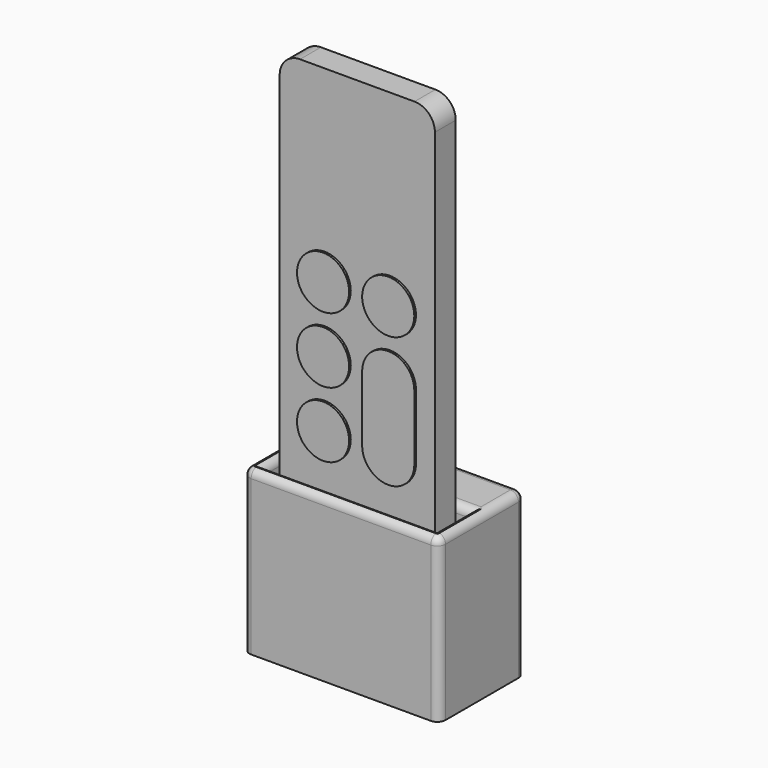
from build123d import *

# Parameters (mm, degrees)
F1_DEPTH      = 6.4
F2_R          = 6.4
F3_DEPTH      = 0.5
F5_DEPTH      = 35
F5_DEPTH_BACK = 5
F6_T          = -3
F7_W          = 48.1
F7_H          = 40
F8_DEPTH      = 10
F9_T1_DEPTH   = 22.4
F9_T3_DEPTH   = 44.1
F9_T5_DEPTH   = 10.4
F9_T7_DEPTH   = 42.1
F9_T9_DEPTH   = 43
F9_S13_W      = 2
F9_S13_H      = 2
F9_T14_DEPTH  = 2
F9_S19_W      = 2
F9_S19_H      = 2
F9_T20_DEPTH  = 2
F9_S25_W      = 2
F9_S25_H      = 2
F9_T26_DEPTH  = 2
F9_S31_W      = 2
F9_S31_H      = 2
F9_T32_DEPTH  = 2
F9_T39_DEPTH  = 15.4
F9_T43_DEPTH  = 47.1
F9_T50_DEPTH  = 15.4
F9_T54_DEPTH  = 47.1
F9_T61_DEPTH  = 47.1
F9_T65_DEPTH  = 15.4
F9_T72_DEPTH  = 15.4
F9_T76_DEPTH  = 47.1


# Not quite as in the source:
# - a fillet or chamfer that OpenCascade refuses, or shapes differently, is made with other operations: its cross-section is extruded or revolved along the edge and cut away or added


with BuildPart() as f1:
    # F0 (on Front) → F1 (new body)
    with BuildSketch(Plane.XZ):
        with BuildLine():
            ThreePointArc((19.05, 57.1), (17.5855339059, 60.6355339059), (14.05, 62.1))
            Line((14.05, 62.1), (-14.05, 62.1))
            ThreePointArc((-14.05, 62.1), (-17.5855339059, 60.6355339059), (-19.05, 57.1))
            Line((-19.05, 57.1), (-19.05, -57.1))
            ThreePointArc((-19.05, -57.1), (-17.5855339059, -60.6355339059), (-14.05, -62.1))
            Line((-14.05, -62.1), (14.05, -62.1))
            ThreePointArc((14.05, -62.1), (17.5855339059, -60.6355339059), (19.05, -57.1))
            Line((19.05, -57.1), (19.05, 57.1))
        make_face()
    extrude(amount=F1_DEPTH)

    # F2 (on face) → F3 (join)
    with BuildSketch(Plane.XZ.offset(6.4)):
        with BuildLine():
            ThreePointArc((1.6, 0), (8, -6.4), (14.4, 0))
            ThreePointArc((14.4, 0), (8, 6.4), (1.6, 0))
        make_face()
        with BuildLine():
            Line((14.4, -16.1), (14.4, 0))
            ThreePointArc((14.4, 0), (8, -6.4), (1.6, 0))
            Line((1.6, 0), (1.6, -16.1))
            ThreePointArc((1.6, -16.1), (8, -9.7), (14.4, -16.1))
        make_face()
        with BuildLine():
            ThreePointArc((1.6, -16.1), (8, -22.5), (14.4, -16.1))
            ThreePointArc((14.4, -16.1), (8, -9.7), (1.6, -16.1))
        make_face()
        with Locations((8, 16.1)):
            Circle(F2_R)
        with Locations((-8, 16.1)):
            Circle(F2_R)
        with Locations((-8, 0)):
            Circle(F2_R)
        with Locations((-8, -16.1)):
            Circle(F2_R)
    extrude(amount=F3_DEPTH)


with BuildPart() as f5:
    # F4 (on face) → F5 (new body, two sides)
    with BuildSketch(Plane(origin=(0, 0, -62.1), x_dir=(1, 0, 0), z_dir=(0, 0, -1))) as f5_sk:
        Polygon((-14.05, 11.4), (-24.05, 11.4), (-24.05, -5), (-14.05, -5), (14.05, -5), (24.05, -5), (24.05, 11.4), (14.05, 11.4), align=None)
    extrude(amount=-F5_DEPTH)
    extrude(f5_sk.sketch, amount=F5_DEPTH_BACK)

    # F6
    f6_openings = [f5.faces().sort_by_distance(p)[0] for p in [
        (0, -3.2, -27.1),
    ]]
    offset(amount=F6_T, openings=f6_openings)

    # F7 (on face) → F8 (join)
    with BuildSketch(Plane(origin=(0, 5, 0), x_dir=(-1, 0, 0), z_dir=(0, 1, 0))):
        with Locations((0, -47.1)):
            Rectangle(F7_W, F7_H)
    extrude(amount=F8_DEPTH)

    # F9: fillet of radius 2 on 12 edges, made by hand

    # F9_s2 → F9_t1 (cut)
    with BuildSketch(Plane.XZ.offset(-13)):
        with BuildLine():
            ThreePointArc((-24.05, -29.1), (-23.4642135624, -27.6857864376), (-22.05, -27.1))
            Line((-22.05, -27.1), (-24.05, -27.1))
            Line((-24.05, -27.1), (-24.05, -29.1))
        make_face()
        with BuildLine():
            ThreePointArc((24.05, -29.1), (23.4642135624, -27.6857864376), (22.05, -27.1))
            Line((22.05, -27.1), (24.05, -27.1))
            Line((24.05, -27.1), (24.05, -29.1))
        make_face()
    extrude(amount=F9_T1_DEPTH, mode=Mode.SUBTRACT)

    # F9_s4 → F9_t3 (cut)
    with BuildSketch(Plane.YZ.offset(-22.05)):
        with BuildLine():
            ThreePointArc((15, -29.1), (14.4142135624, -27.6857864376), (13, -27.1))
            Line((13, -27.1), (15, -27.1))
            Line((15, -27.1), (15, -29.1))
        make_face()
        with BuildLine():
            ThreePointArc((-11.4, -29.1), (-10.8142135624, -27.6857864376), (-9.4, -27.1))
            Line((-9.4, -27.1), (-11.4, -27.1))
            Line((-11.4, -27.1), (-11.4, -29.1))
        make_face()
    extrude(amount=F9_T3_DEPTH, mode=Mode.SUBTRACT)

    # F9_s6 → F9_t5 (cut)
    with BuildSketch(Plane.XZ.offset(-2)):
        with BuildLine():
            ThreePointArc((-23.05, -27.1), (-21.6357864376, -27.6857864376), (-21.05, -29.1))
            Line((-21.05, -29.1), (-21.05, -27.1))
            Line((-21.05, -27.1), (-23.05, -27.1))
        make_face()
        with BuildLine():
            ThreePointArc((23.05, -27.1), (21.6357864376, -27.6857864376), (21.05, -29.1))
            Line((21.05, -29.1), (21.05, -27.1))
            Line((21.05, -27.1), (23.05, -27.1))
        make_face()
    extrude(amount=F9_T5_DEPTH, mode=Mode.SUBTRACT)

    # F9_s8 → F9_t7 (cut)
    with BuildSketch(Plane.YZ.offset(-21.05)):
        with BuildLine():
            ThreePointArc((-10.4, -27.1), (-8.9857864376, -27.6857864376), (-8.4, -29.1))
            Line((-8.4, -29.1), (-8.4, -27.1))
            Line((-8.4, -27.1), (-10.4, -27.1))
        make_face()
        with BuildLine():
            ThreePointArc((4, -27.1), (2.5857864376, -27.6857864376), (2, -29.1))
            Line((2, -29.1), (2, -27.1))
            Line((2, -27.1), (4, -27.1))
        make_face()
    extrude(amount=F9_T7_DEPTH, mode=Mode.SUBTRACT)

    # F9_s10 → F9_t9 (cut)
    with BuildSketch(Plane.XY.offset(-72.1)):
        with BuildLine():
            ThreePointArc((22.05, -11.4), (23.4642135624, -10.8142135624), (24.05, -9.4))
            Line((24.05, -9.4), (24.05, -11.4))
            Line((24.05, -11.4), (22.05, -11.4))
        make_face()
        with BuildLine():
            ThreePointArc((24.05, 13), (23.4642135624, 14.4142135624), (22.05, 15))
            Line((22.05, 15), (24.05, 15))
            Line((24.05, 15), (24.05, 13))
        make_face()
        with BuildLine():
            ThreePointArc((-22.05, 15), (-23.4642135624, 14.4142135624), (-24.05, 13))
            Line((-24.05, 13), (-24.05, 15))
            Line((-24.05, 15), (-22.05, 15))
        make_face()
        with BuildLine():
            ThreePointArc((-22.05, -11.4), (-23.4642135624, -10.8142135624), (-24.05, -9.4))
            Line((-24.05, -9.4), (-24.05, -11.4))
            Line((-24.05, -11.4), (-22.05, -11.4))
        make_face()
    extrude(amount=F9_T9_DEPTH, mode=Mode.SUBTRACT)


with BuildPart() as f9_tool12:
    # F9_s13 → F9_t14 (new body)
    with BuildSketch(Plane.XZ.offset(-13)):
        with Locations((-23.05, -28.1)):
            Rectangle(F9_S13_W, F9_S13_H)
    extrude(amount=-F9_T14_DEPTH)

    # F9_s15 → F9_t16 (revolve, cut)
    with BuildSketch(Plane(origin=(-22.05, 13, -29.1), x_dir=(0.7071067812, 0, -0.7071067812), z_dir=(0.7071067812, 0, 0.7071067812))):
        with BuildLine():
            ThreePointArc((0, -2), (2, 0), (0, 2))
            Line((0, 2), (0, -2))
        make_face()
    revolve(axis=Axis((-22.05, 13, -29.1), (0, 1, 0)), mode=Mode.SUBTRACT)


with BuildPart() as f5_1:
    add(f5.part)

    # F9_t11: cut F9_tool12
    add(f9_tool12.part, mode=Mode.SUBTRACT)


with BuildPart() as f9_tool18:
    # F9_s19 → F9_t20 (new body)
    with BuildSketch(Plane.XZ.offset(9.4)):
        with Locations((-23.05, -28.1)):
            Rectangle(F9_S19_W, F9_S19_H)
    extrude(amount=F9_T20_DEPTH)

    # F9_s21 → F9_t22 (revolve, cut)
    with BuildSketch(Plane(origin=(-22.05, -9.4, -29.1), x_dir=(0.7071067812, 0, -0.7071067812), z_dir=(-0.7071067812, 0, -0.7071067812))):
        with BuildLine():
            ThreePointArc((0, -2), (2, 0), (0, 2))
            Line((0, 2), (0, -2))
        make_face()
    revolve(axis=Axis((-22.05, -9.4, -29.1), (0, -1, 0)), mode=Mode.SUBTRACT)


with BuildPart() as f5_2:
    add(f5_1.part)

    # F9_t17: cut F9_tool18
    add(f9_tool18.part, mode=Mode.SUBTRACT)


with BuildPart() as f9_tool24:
    # F9_s25 → F9_t26 (new body)
    with BuildSketch(Plane.YZ.offset(22.05)):
        with Locations((14, -28.1)):
            Rectangle(F9_S25_W, F9_S25_H)
    extrude(amount=F9_T26_DEPTH)

    # F9_s27 → F9_t28 (revolve, cut)
    with BuildSketch(Plane(origin=(22.05, 13, -29.1), x_dir=(0, -0.7071067812, -0.7071067812), z_dir=(0, -0.7071067812, 0.7071067812))):
        with BuildLine():
            ThreePointArc((0, -2), (2, 0), (0, 2))
            Line((0, 2), (0, -2))
        make_face()
    revolve(axis=Axis((22.05, 13, -29.1), (1, 0, 0)), mode=Mode.SUBTRACT)


with BuildPart() as f5_3:
    add(f5_2.part)

    # F9_t23: cut F9_tool24
    add(f9_tool24.part, mode=Mode.SUBTRACT)


with BuildPart() as f9_tool30:
    # F9_s31 → F9_t32 (new body)
    with BuildSketch(Plane.XZ.offset(9.4)):
        with Locations((23.05, -28.1)):
            Rectangle(F9_S31_W, F9_S31_H)
    extrude(amount=F9_T32_DEPTH)

    # F9_s33 → F9_t34 (revolve, cut)
    with BuildSketch(Plane(origin=(22.05, -9.4, -29.1), x_dir=(-0.7071067812, 0, -0.7071067812), z_dir=(-0.7071067812, 0, 0.7071067812))):
        with BuildLine():
            ThreePointArc((0, -2), (2, 0), (0, 2))
            Line((0, 2), (0, -2))
        make_face()
    revolve(axis=Axis((22.05, -9.4, -29.1), (0, -1, 0)), mode=Mode.SUBTRACT)


with BuildPart() as f5_4:
    add(f5_3.part)

    # F9_t29: cut F9_tool30
    add(f9_tool30.part, mode=Mode.SUBTRACT)


with BuildPart() as f9_tool37:
    # F9_s38 → F9_t39 (new body)
    with BuildSketch(Plane.XZ.offset(13.4)):
        with BuildLine():
            ThreePointArc((-23.05, -27.1), (-21.6357864376, -27.6857864376), (-21.05, -29.1))
            Line((-21.05, -29.1), (-21.05, -27.1))
            Line((-21.05, -27.1), (-23.05, -27.1))
        make_face()
    extrude(amount=-F9_T39_DEPTH)

    split(bisect_by=Plane.XZ.offset(8.4), keep=Keep.TOP)


with BuildPart() as f9_tool41:
    # F9_s42 → F9_t43 (new body)
    with BuildSketch(Plane.YZ.offset(21.05)):
        with BuildLine():
            ThreePointArc((-10.4, -27.1), (-8.9857864376, -27.6857864376), (-8.4, -29.1))
            Line((-8.4, -29.1), (-8.4, -27.1))
            Line((-8.4, -27.1), (-10.4, -27.1))
        make_face()
    extrude(amount=-F9_T43_DEPTH)

    split(bisect_by=Plane.YZ.offset(-21.05), keep=Keep.BOTTOM)


with BuildPart() as f9_tool37_1:
    add(f9_tool37.part)

    # F9_t45: intersect F9_tool41
    add(f9_tool41.part, mode=Mode.INTERSECT)


with BuildPart() as f5_5:
    add(f5_4.part)

    # F9_t35: cut F9_tool37
    add(f9_tool37_1.part, mode=Mode.SUBTRACT)


with BuildPart() as f9_tool48:
    # F9_s49 → F9_t50 (new body)
    with BuildSketch(Plane.XZ.offset(8.4)):
        with BuildLine():
            ThreePointArc((-23.05, -27.1), (-21.6357864376, -27.6857864376), (-21.05, -29.1))
            Line((-21.05, -29.1), (-21.05, -27.1))
            Line((-21.05, -27.1), (-23.05, -27.1))
        make_face()
    extrude(amount=-F9_T50_DEPTH)

    split(bisect_by=Plane.XZ.offset(-2), keep=Keep.BOTTOM)


with BuildPart() as f9_tool52:
    # F9_s53 → F9_t54 (new body)
    with BuildSketch(Plane.YZ.offset(-26.05)):
        with BuildLine():
            ThreePointArc((4, -27.1), (2.5857864376, -27.6857864376), (2, -29.1))
            Line((2, -29.1), (2, -27.1))
            Line((2, -27.1), (4, -27.1))
        make_face()
    extrude(amount=F9_T54_DEPTH)

    split(bisect_by=Plane.YZ.offset(-21.05), keep=Keep.BOTTOM)


with BuildPart() as f9_tool48_1:
    add(f9_tool48.part)

    # F9_t56: intersect F9_tool52
    add(f9_tool52.part, mode=Mode.INTERSECT)


with BuildPart() as f5_6:
    add(f5_5.part)

    # F9_t46: cut F9_tool48
    add(f9_tool48_1.part, mode=Mode.SUBTRACT)


with BuildPart() as f9_tool59:
    # F9_s60 → F9_t61 (new body)
    with BuildSketch(Plane.YZ.offset(26.05)):
        with BuildLine():
            ThreePointArc((-10.4, -27.1), (-8.9857864376, -27.6857864376), (-8.4, -29.1))
            Line((-8.4, -29.1), (-8.4, -27.1))
            Line((-8.4, -27.1), (-10.4, -27.1))
        make_face()
    extrude(amount=-F9_T61_DEPTH)

    split(bisect_by=Plane.YZ.offset(21.05), keep=Keep.TOP)


with BuildPart() as f9_tool63:
    # F9_s64 → F9_t65 (new body)
    with BuildSketch(Plane.XZ.offset(-2)):
        with BuildLine():
            ThreePointArc((23.05, -27.1), (21.6357864376, -27.6857864376), (21.05, -29.1))
            Line((21.05, -29.1), (21.05, -27.1))
            Line((21.05, -27.1), (23.05, -27.1))
        make_face()
    extrude(amount=F9_T65_DEPTH)

    split(bisect_by=Plane.XZ.offset(8.4), keep=Keep.TOP)


with BuildPart() as f9_tool59_1:
    add(f9_tool59.part)

    # F9_t67: intersect F9_tool63
    add(f9_tool63.part, mode=Mode.INTERSECT)


with BuildPart() as f5_7:
    add(f5_6.part)

    # F9_t57: cut F9_tool59
    add(f9_tool59_1.part, mode=Mode.SUBTRACT)


with BuildPart() as f9_tool70:
    # F9_s71 → F9_t72 (new body)
    with BuildSketch(Plane.XZ.offset(-7)):
        with BuildLine():
            ThreePointArc((23.05, -27.1), (21.6357864376, -27.6857864376), (21.05, -29.1))
            Line((21.05, -29.1), (21.05, -27.1))
            Line((21.05, -27.1), (23.05, -27.1))
        make_face()
    extrude(amount=F9_T72_DEPTH)

    split(bisect_by=Plane.XZ.offset(-2), keep=Keep.BOTTOM)


with BuildPart() as f9_tool74:
    # F9_s75 → F9_t76 (new body)
    with BuildSketch(Plane.YZ.offset(-21.05)):
        with BuildLine():
            ThreePointArc((4, -27.1), (2.5857864376, -27.6857864376), (2, -29.1))
            Line((2, -29.1), (2, -27.1))
            Line((2, -27.1), (4, -27.1))
        make_face()
    extrude(amount=F9_T76_DEPTH)

    split(bisect_by=Plane.YZ.offset(21.05), keep=Keep.TOP)


with BuildPart() as f9_tool70_1:
    add(f9_tool70.part)

    # F9_t78: intersect F9_tool74
    add(f9_tool74.part, mode=Mode.INTERSECT)


with BuildPart() as f5_8:
    add(f5_7.part)

    # F9_t68: cut F9_tool70
    add(f9_tool70_1.part, mode=Mode.SUBTRACT)


solid = Compound([f1.part, f5_8.part])
